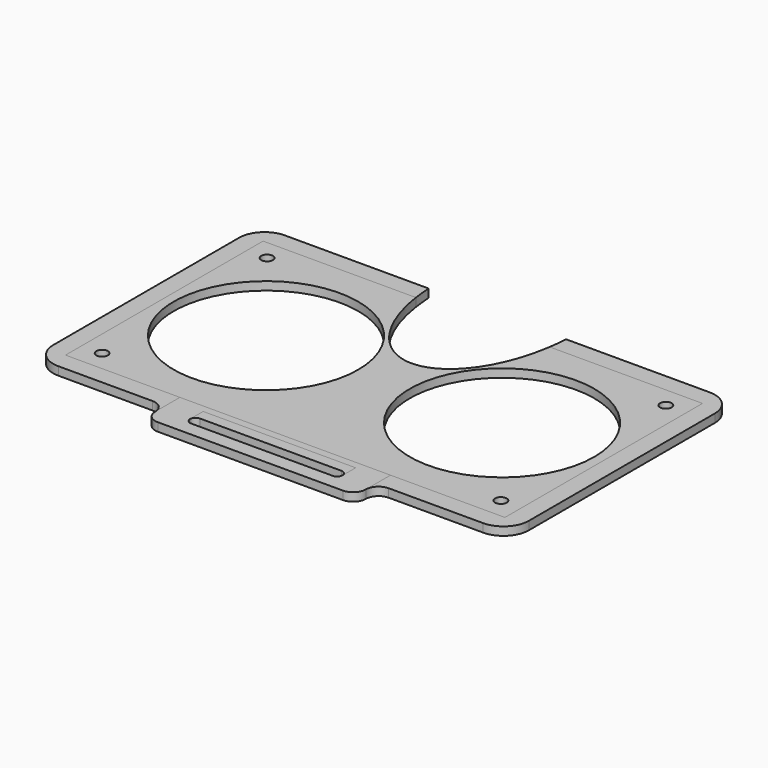
from build123d import *

# Parameters (mm, degrees)
F3_DEPTH = 2.3
F0_W     = 121
F0_H     = 68
F0_R     = 1.6
F0_R_2   = 25.4
F4_DEPTH = 25
F6_DEPTH = 2.3
F1_W     = 42
F1_H     = 3
F7_DEPTH = 2.3
F8_R     = 7
F9_R     = 3.49999
F10_R    = 1.49999


# Not quite as in the source:
# - a fillet or chamfer is up to 0.001 mm smaller than in the source, because OpenCascade refuses the exact size


with BuildPart() as f3:
    # F2 (on face) → F3 (new body)
    with BuildSketch(Plane.XY):
        with BuildLine():
            add(Edge.make_bspline(
                [(18.4153846154, 34), (18.7815631387, 36.4662846266), (18.9188800849, 39)],
                knots=[1.3220863377, 1.3220863377, 1.3220863377, 1.4783570414, 1.4783570414, 1.4783570414], degree=2, weights=[1, 0.9969489861, 1]))
            Line((18.4153846154, 34), (60.5, 34))
            Line((60.5, 34), (60.5, -34))
            Line((60.5, -34), (29, -34))
            Line((29, -34), (29, -39))
            Line((29, -39), (65.5, -39))
            Line((65.5, -39), (65.5, 39))
            Line((65.5, 39), (18.9188800849, 39))
        make_face()
    extrude(amount=F3_DEPTH)


with BuildPart() as f3b:
    # F2 (on face) → F3, piece 2 (new body)
    with BuildSketch(Plane.XY):
        with BuildLine():
            Line((-60.5, 34), (-18.4153846154, 34))
            add(Edge.make_bspline(
                [(-18.9188800849, 39), (-18.7815631387, 36.4662846266), (-18.4153846154, 34)],
                knots=[4.8048282657, 4.8048282657, 4.8048282657, 4.9610989695, 4.9610989695, 4.9610989695], degree=2, weights=[1, 0.9969489861, 1]))
            Line((-18.9188800849, 39), (-65.5, 39))
            Line((-65.5, 39), (-65.5, -39))
            Line((-65.5, -39), (-29, -39))
            Line((-29, -39), (-29, -34))
            Line((-29, -34), (-60.5, -34))
            Line((-60.5, -34), (-60.5, 34))
        make_face()
    extrude(amount=F3_DEPTH)


with BuildPart() as f3c:
    # F0 (on Top) → F3, piece 3 (new body)
    with BuildSketch(Plane.XY):
        Rectangle(F0_W, F0_H)
        with Locations((-54.9, -28.4)):
            Circle(F0_R, mode=Mode.SUBTRACT)
        with Locations((54.9, -28.4)):
            Circle(F0_R, mode=Mode.SUBTRACT)
        with Locations((-32.5, 0)):
            Circle(F0_R_2, mode=Mode.SUBTRACT)
        with Locations((-54.9, 28.4)):
            Circle(F0_R, mode=Mode.SUBTRACT)
        with Locations((32.5, 0)):
            Circle(F0_R_2, mode=Mode.SUBTRACT)
        with Locations((54.9, 28.4)):
            Circle(F0_R, mode=Mode.SUBTRACT)
    extrude(amount=F3_DEPTH)

    # F2 (on face) → F4 (cut)
    with BuildSketch(Plane.XY):
        with BuildLine():
            add(Edge.make_bspline(
                [(0, 9.5), (32.9089653438, 9.5), (16.4544826719, 58.25), (0, 107), (-16.4544826719, 58.25), (-32.9089653438, 9.5), (0, 9.5)],
                knots=[0, 0, 0, 2.0943951024, 2.0943951024, 4.1887902048, 4.1887902048, 6.2831853072, 6.2831853072, 6.2831853072], degree=2, weights=[1, 0.5, 1, 0.5, 1, 0.5, 1]))
        make_face()
    extrude(amount=F4_DEPTH, mode=Mode.SUBTRACT)

    # F5: union F3, F3b
    add(f3.part)
    add(f3b.part)

    # F1 (on Top) → F6 (join, through all)
    with BuildSketch(Plane.XY):
        Polygon((29, -39), (29, -34), (-29, -34), (-29, -39), (-21, -39), (-21, -36), (21, -36), (21, -39), align=None)
        Polygon((29, -46), (29, -39), (21, -39), (21, -42), (-21, -42), (-21, -39), (-29, -39), (-29, -46), align=None)
    extrude(amount=F6_DEPTH)

    # F1 (on Top) → F7 (join, through all)
    with BuildSketch(Plane.XY):
        with Locations((0, -37.5)):
            Rectangle(F1_W, F1_H)
    extrude(amount=F7_DEPTH)

    # F8
    f8_edges = [f3c.edges().sort_by_distance(p)[0] for p in [
        (65.5, -39, 1.15),
        (65.5, 39, 1.15),
        (-65.5, 39, 1.15),
        (-65.5, -39, 1.15),
    ]]
    fillet(f8_edges, radius=F8_R)

    # F9 (radius 3.5 in the source; OpenCascade refuses exactly that, so slightly less here)
    f9_edges = [f3c.edges().sort_by_distance(p)[0] for p in [
        (29, -39, 1.15),
        (29, -46, 1.15),
        (-29, -39, 1.15),
        (-29, -46, 1.15),
    ]]
    fillet(f9_edges, radius=F9_R)

    # F10 (radius 1.5 in the source; OpenCascade refuses exactly that, so slightly less here)
    f10_edges = [f3c.edges().sort_by_distance(p)[0] for p in [
        (-21, -42, 1.15),
        (-21, -39, 1.15),
        (21, -42, 1.15),
        (21, -39, 1.15),
    ]]
    fillet(f10_edges, radius=F10_R)


solid = f3c.part
